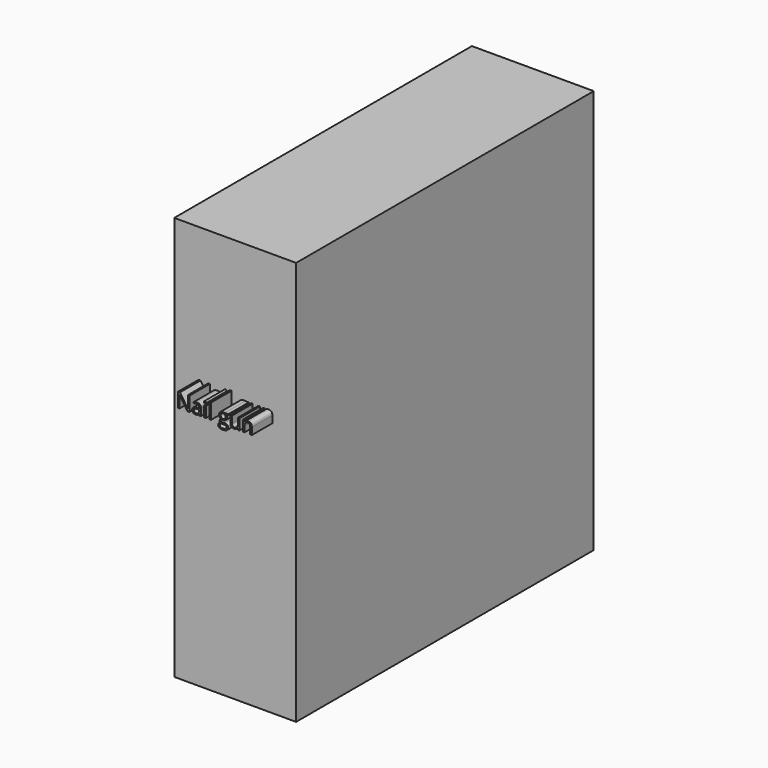
from build123d import *

# Parameters (mm, degrees)
F0_W         = 120.65
F0_H         = 400.05
F1_DEPTH     = 368.3
F2_TEXT_SIZE = 19.8671935471
F3_DEPTH     = 25.4


# Not quite as in the source:
# - Text() gives the source's letters only with a copy of the font that has no kerning and outlines rounded to 1/6400 em; it was checked with that copy


with BuildPart() as f1:
    # F0 (on Front) → F1 (new body)
    with BuildSketch(Plane.XZ):
        Rectangle(F0_W, F0_H)
    extrude(amount=F1_DEPTH)

    # F2 (on face) → F3 (join)
    with BuildSketch(Plane.XZ.offset(368.3)):
        with Locations((-38.1, 52.6256880383)):
            Text('Nail gun', F2_TEXT_SIZE, font='Open Sans', text_align=(TextAlign.LEFT, TextAlign.BOTTOM))
    extrude(amount=F3_DEPTH)


solid = f1.part
